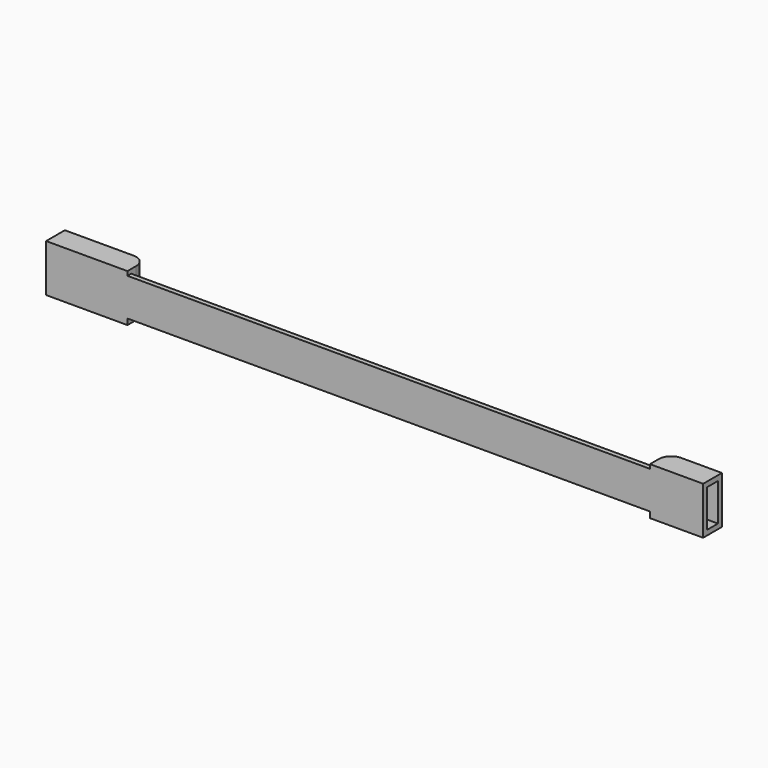
from build123d import *

# Parameters (mm, degrees)
F3_W          = 7.5
F3_H          = 15.2
F5_DEPTH      = 17
F4_W          = 7.5
F4_H          = 15.2
F6_DEPTH      = 26
F0_W          = 200
F0_H          = 12
F7_DEPTH      = 1.5
F8_W          = 4.3
F8_H          = 12
F9_DEPTH      = 14
F10_W         = 4.3
F10_H         = 12
F11_DEPTH     = 22.5
F12_TEXT_SIZE = 9.3315983476
F13_DEPTH     = 1
F14_R         = 4
F14_2_R       = 4
F16_TEXT_SIZE = 11.1111111111
F17_DEPTH     = 1
F18_R         = 1.5
F19_DEPTH     = 5


# Not quite as in the source:
# - a feature names something its author has since deleted; it is built from what else it names
# - Text() gives the source's letters only with a copy of the font that has no kerning and outlines rounded to 1/6400 em; it was checked with that copy


with BuildPart() as f5:
    # F3 (on offset) → F5 (new body)
    with BuildSketch(Plane.YZ.offset(105)):
        with Locations((3.75, 3.85)):
            Rectangle(F3_W, F3_H)
    extrude(amount=-F5_DEPTH)

    # F8 (on offset) → F9 (cut)
    with BuildSketch(Plane.YZ.offset(105)):
        with Locations((3.75, 3.85)):
            Rectangle(F8_W, F8_H)
    extrude(amount=-F9_DEPTH, mode=Mode.SUBTRACT)

    # F14#2
    f14_2_edges = [f5.edges().sort_by_distance(p)[0] for p in [
        (88, 7.5, 3.85),
    ]]
    fillet(f14_2_edges, radius=F14_2_R)


with BuildPart() as f6:
    # F4 (on offset) → F6 (new body)
    with BuildSketch(Plane.YZ.offset(-105)):
        with Locations((3.75, 3.85)):
            Rectangle(F4_W, F4_H)
    extrude(amount=F6_DEPTH)

    # F10 (on offset) → F11 (cut)
    with BuildSketch(Plane.YZ.offset(-105)):
        with Locations((3.75, 3.85)):
            Rectangle(F10_W, F10_H)
    extrude(amount=F11_DEPTH, mode=Mode.SUBTRACT)

    # F14
    f14_edges = [f6.edges().sort_by_distance(p)[0] for p in [
        (-79, 7.5, 3.85),
    ]]
    fillet(f14_edges, radius=F14_R)


with BuildPart() as f7:
    # F0 (on Front) → F7 (new body)
    with BuildSketch(Plane.XZ):
        with Locations((0, 4.125)):
            Rectangle(F0_W, F0_H)
    extrude(amount=-F7_DEPTH)

    # F12 (on face) → F13 (join)
    with BuildSketch(Plane(origin=(0, 1.5, 0), x_dir=(-1, 0, 0), z_dir=(0, 1, 0))):
        with Locations((-23.051964043, 0.7992716855)):
            Text('IES de Teis', F12_TEXT_SIZE, font='Open Sans', text_align=(TextAlign.LEFT, TextAlign.BOTTOM))
    extrude(amount=F13_DEPTH)


with BuildPart() as f5_1:
    add(f5.part)

    # F15: union F6, F7
    add(f6.part)
    add(f7.part)

    # F16 (on face) → F17 (join)
    with BuildSketch(Plane(origin=(0, 7.5, 0), x_dir=(-1, 0, 0), z_dir=(0, 1, 0))):
        with Locations(Location((83.0004177496, -0.1499999891), (0, 0, 0.0029919111))):
            Text('SFS', F16_TEXT_SIZE, font='Open Sans', text_align=(TextAlign.LEFT, TextAlign.BOTTOM))
    extrude(amount=F17_DEPTH)

    # F18 (on face) → F19 (join)
    with BuildSketch(Plane.XZ):
        with Locations((-87.5, 3.85)):
            Circle(F18_R)
    extrude(amount=-F19_DEPTH)


solid = f5_1.part
